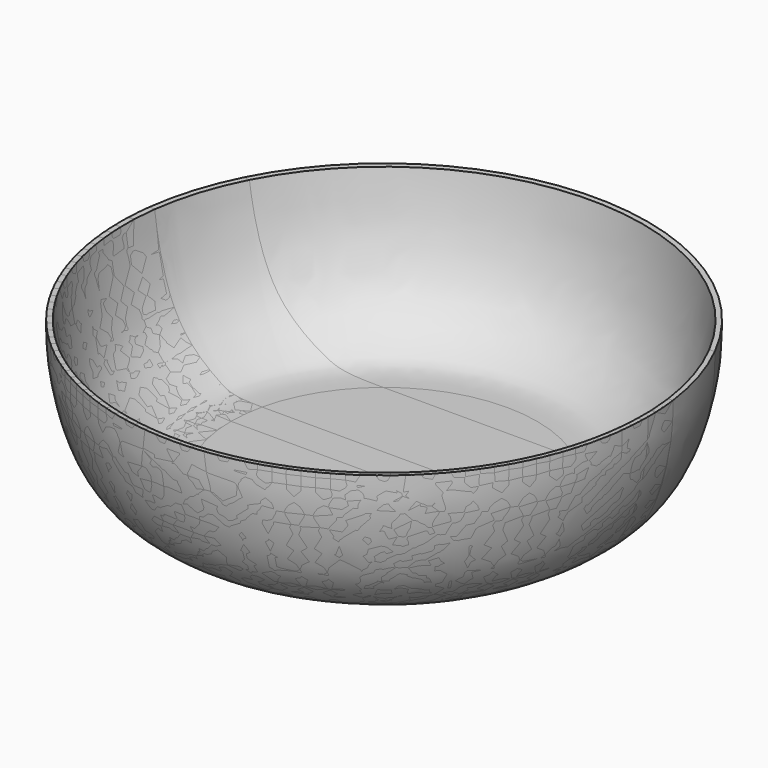
from build123d import *

# Parameters (mm, degrees)
F1_DEPTH  = 50
F2_DEPTH  = 50
F3_DEPTH  = 50
F4_DEPTH  = 50
F5_DEPTH  = 50
F6_DEPTH  = 50
F7_DEPTH  = 50
F8_DEPTH  = 50
F9_DEPTH  = 50
F10_DEPTH = 50
F11_DEPTH = 50
F12_DEPTH = 50


# Not quite as in the source:
# - a feature names something its author has since deleted; it is built from what else it names


with BuildPart() as f1:
    # F0 (on Top) → F1 (new body)
    with BuildSketch(Plane.XY):
        Polygon((0, 70), (0, 25), (90, 25), (115, 25), (160, 25), (160, 70), (115, 70), (90, 70), align=None)
    extrude(amount=F1_DEPTH)


with BuildPart() as f2:
    # F0 (on Top) → F2 (new body)
    with BuildSketch(Plane.XY):
        Polygon((0, 70), (0, 25), (90, 25), (115, 25), (160, 25), (160, 70), (115, 70), (90, 70), align=None)
    extrude(amount=F2_DEPTH)


with BuildPart() as f3:
    # F0 (on Top) → F3 (new body)
    with BuildSketch(Plane.XY):
        Polygon((0, 70), (0, 25), (90, 25), (115, 25), (160, 25), (160, 70), (115, 70), (90, 70), align=None)
    extrude(amount=F3_DEPTH)


with BuildPart() as f4:
    # F0 (on Top) → F4 (new body)
    with BuildSketch(Plane.XY):
        Polygon((0, 25), (0, 0), (90, 0), (100, 0), (115, 0), (125, 0), (160, 0), (160, 25), (115, 25), (90, 25), align=None)
    extrude(amount=F4_DEPTH)


with BuildPart() as f5:
    # F0 (on Top) → F5 (new body)
    with BuildSketch(Plane.XY):
        Polygon((90, 0), (0, 0), (0, -10), (160, -10), (160, 0), (125, 0), (115, 0), (100, 0), align=None)
        Polygon((160, -10), (0, -10), (0, -90), (90, -90), (115, -90), (160, -90), align=None)
    extrude(amount=F5_DEPTH)


with BuildPart() as f6:
    # F0 (on Top) → F6 (new body)
    with BuildSketch(Plane.XY):
        Polygon((90, 0), (0, 0), (0, -10), (160, -10), (160, 0), (125, 0), (115, 0), (100, 0), align=None)
        Polygon((160, -10), (0, -10), (0, -90), (90, -90), (115, -90), (160, -90), align=None)
    extrude(amount=F6_DEPTH)


with BuildPart() as f7:
    # F0 (on Top) → F7 (new body)
    with BuildSketch(Plane.XY):
        Polygon((90, 0), (0, 0), (0, -10), (160, -10), (160, 0), (125, 0), (115, 0), (100, 0), align=None)
    extrude(amount=F7_DEPTH)


with BuildPart() as f8:
    # F0 (on Top) → F8 (new body)
    with BuildSketch(Plane.XY):
        Polygon((90, 0), (0, 0), (0, -10), (160, -10), (160, 0), (125, 0), (115, 0), (100, 0), align=None)
    extrude(amount=F8_DEPTH)


with BuildPart() as f9:
    # F0 (on Top) → F9 (new body)
    with BuildSketch(Plane.XY):
        Polygon((90, 0), (0, 0), (0, -10), (160, -10), (160, 0), (125, 0), (115, 0), (100, 0), align=None)
    extrude(amount=F9_DEPTH)


with BuildPart() as f10:
    # F0 (on Top) → F10 (new body)
    with BuildSketch(Plane.XY):
        Polygon((160, -10), (0, -10), (0, -90), (90, -90), (115, -90), (160, -90), align=None)
    extrude(amount=F10_DEPTH)


with BuildPart() as f11:
    # F0 (on Top) → F11 (new body)
    with BuildSketch(Plane.XY):
        Polygon((160, -10), (0, -10), (0, -90), (90, -90), (115, -90), (160, -90), align=None)
    extrude(amount=F11_DEPTH)


with BuildPart() as f12:
    # F0 (on Top) → F12 (new body)
    with BuildSketch(Plane.XY):
        Polygon((160, -10), (0, -10), (0, -90), (90, -90), (115, -90), (160, -90), align=None)
    extrude(amount=F12_DEPTH)


with BuildPart() as f14_tool:
    # F13 (on face) → F14 (revolve)
    with BuildSketch(Plane.XZ.offset(10)):
        with BuildLine():
            Line((80, 8.0908760428), (80, 4))
            Line((80, 4), (106, 4))
            Line((106, 4), (104.1045635939, 0))
            Line((104.1045635939, 0), (119.1045635939, 0))
            add(Edge.make_bspline(
                [(119.1045635939, 0), (126.7783361131, 0.9991904563), (131.3802074289, 2.1137068882), (151.3517987192, 11.4378454195), (157.3482452654, 37.4682067973), (157.5913219248, 44.137306747), (157.5940996408, 49.1173379123)],
                knots=[0, 0, 0, 0, 0.2254306691, 0.4876229216, 0.7876886563, 1, 1, 1, 1], degree=3))
            Line((157.5940996408, 49.1173379123), (156.1105251312, 49.0066148341))
            add(Edge.make_bspline(
                [(125, 8.0908760428), (133.0497704804, 8.0908760428), (136.3638110844, 9.6508818987), (151.6141774336, 21.42212707), (155.1475136349, 40.8154585524), (156.1105251312, 49.0066148341)],
                knots=[0, 0, 0, 0, 0.2773229228, 0.5906271351, 1, 1, 1, 1], degree=3))
            Line((125, 8.0908760428), (80, 8.0908760428))
        make_face()
    revolve(axis=Axis((80, -10, 22.4669491872), (0, 0, -1)))


with BuildPart() as f1_1:
    add(f1.part)

    # F14: intersect by f14_tool
    add(f14_tool.part, mode=Mode.INTERSECT)


with BuildPart() as f2_1:
    add(f2.part)

    # F14: intersect by f14_tool
    add(f14_tool.part, mode=Mode.INTERSECT)


with BuildPart() as f3_1:
    add(f3.part)

    # F14: intersect by f14_tool
    add(f14_tool.part, mode=Mode.INTERSECT)


with BuildPart() as f4_1:
    add(f4.part)

    # F14: intersect by f14_tool
    add(f14_tool.part, mode=Mode.INTERSECT)


with BuildPart() as f5_1:
    add(f5.part)

    # F14: intersect by f14_tool
    add(f14_tool.part, mode=Mode.INTERSECT)


with BuildPart() as f6_1:
    add(f6.part)

    # F14: intersect by f14_tool
    add(f14_tool.part, mode=Mode.INTERSECT)


with BuildPart() as f7_1:
    add(f7.part)

    # F14: intersect by f14_tool
    add(f14_tool.part, mode=Mode.INTERSECT)


with BuildPart() as f8_1:
    add(f8.part)

    # F14: intersect by f14_tool
    add(f14_tool.part, mode=Mode.INTERSECT)


with BuildPart() as f9_1:
    add(f9.part)

    # F14: intersect by f14_tool
    add(f14_tool.part, mode=Mode.INTERSECT)


with BuildPart() as f10_1:
    add(f10.part)

    # F14: intersect by f14_tool
    add(f14_tool.part, mode=Mode.INTERSECT)


with BuildPart() as f11_1:
    add(f11.part)

    # F14: intersect by f14_tool
    add(f14_tool.part, mode=Mode.INTERSECT)


with BuildPart() as f12_1:
    add(f12.part)

    # F14: intersect by f14_tool
    add(f14_tool.part, mode=Mode.INTERSECT)


solid = Compound([f1_1.part, f2_1.part, f3_1.part, f4_1.part, f5_1.part, f6_1.part, f7_1.part, f8_1.part, f9_1.part, f10_1.part, f11_1.part, f12_1.part])
